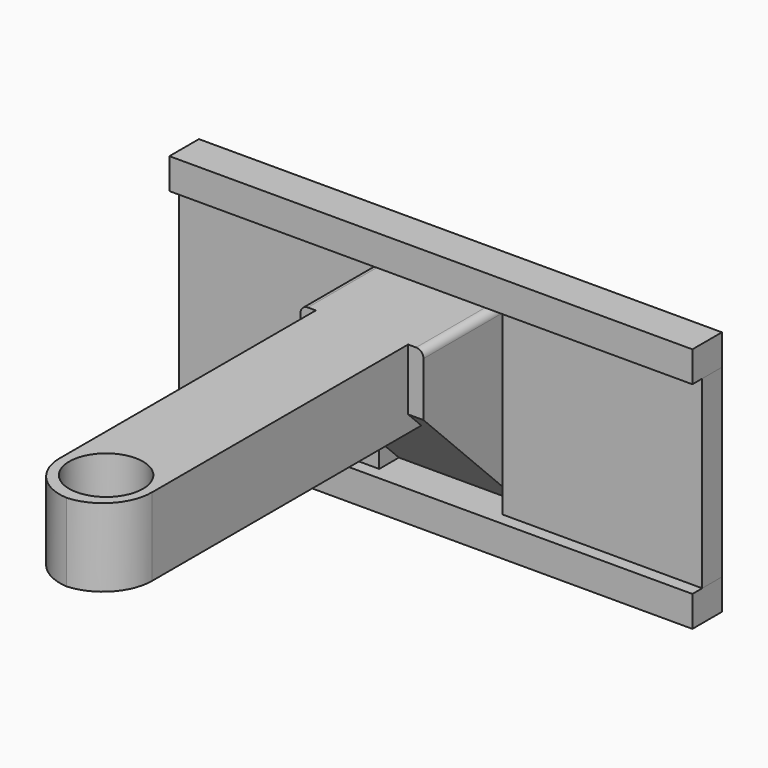
from build123d import *

# Parameters (mm, degrees)
F0_W         = 15.24
F0_H         = 12.7
F0_H_2       = 0.8601994222
F1_DEPTH     = 101.6
F2_DEPTH     = 25.4
F4_START     = 6.35
F3_R         = 7.62
F4_DEPTH     = 18.796
F5_T1_DEPTH  = 66.9001994222
F0_W_2       = 41.275
F0_H_3       = 38.1
F6_DEPTH     = 5.08
F0_W_3       = 107.95
F0_H_4       = 1.016
F0_H_5       = 4.318
F7_DEPTH     = 7.62
F8_R         = 1.524
F9_T4_DEPTH  = 156.0414957887
F9_T10_DEPTH = 156.0414957887
F9_T16_DEPTH = 156.0414957887
F9_T23_DEPTH = 156.0414957887
F9_T29_DEPTH = 156.0414957887


# Not quite as in the source:
# - a fillet or chamfer that OpenCascade refuses, or shapes differently, is made with other operations: its cross-section is extruded or revolved along the edge and cut away or added


with BuildPart() as f1:
    # F0 (on Front) → F1 (new body)
    with BuildSketch(Plane.XZ):
        Polygon((9.525, 2.9498005778), (9.525, 19.05), (7.62, 19.05), (7.62, 18.1898005778), (7.62, 5.4898005778), (-7.62, 5.4898005778), (-7.62, 18.1898005778), (-7.62, 19.05), (-9.525, 19.05), (-9.525, 2.9498005778), align=None)
        with Locations((0, 11.8398005778)):
            Rectangle(F0_W, F0_H)
        with Locations((0, 18.6199002889)):
            Rectangle(F0_W, F0_H_2)
    extrude(amount=F1_DEPTH)

    # F0 (on Front) → F2 (join)
    with BuildSketch(Plane.XZ):
        Polygon((12.7, -19.05), (12.7, 19.05), (9.525, 19.05), (9.525, 2.9498005778), (-9.525, 2.9498005778), (-9.525, 19.05), (-12.7, 19.05), (-12.7, -19.05), align=None)
    extrude(amount=F2_DEPTH)

    # F3 (on Top) → F4 (cut)
    with BuildSketch(Plane.XY.offset(F4_START)):
        with Locations((0, -91.4209560153)):
            Circle(F3_R)
    extrude(amount=F4_DEPTH, mode=Mode.SUBTRACT)

    # F5: fillet of radius 10.16 on 2 edges, made by hand

    # F5_s2 → F5_t1 (cut)
    with BuildSketch(Plane.XY.offset(-22.4501994222)):
        with BuildLine():
            ThreePointArc((9.525, -91.44), (6.5492048969, -98.6242048969), (-0.635, -101.6))
            Line((-0.635, -101.6), (9.525, -101.6))
            Line((9.525, -101.6), (9.525, -91.44))
        make_face()
        with BuildLine():
            ThreePointArc((0.635, -101.6), (-6.5492048969, -98.6242048969), (-9.525, -91.44))
            Line((-9.525, -91.44), (-9.525, -101.6))
            Line((-9.525, -101.6), (0.635, -101.6))
        make_face()
    extrude(amount=F5_T1_DEPTH, mode=Mode.SUBTRACT)

    # F8
    f8_edges = [f1.edges().sort_by_distance(p)[0] for p in [
        (-12.7, -12.7, 19.05),
        (12.7, -12.7, 19.05),
    ]]
    fillet(f8_edges, radius=F8_R)

    # F9: chamfer of 25.4 on 1 edges, made by hand


with BuildPart() as f6:
    # F0 (on Front) → F6 (new body)
    with BuildSketch(Plane.XZ):
        with Locations((-33.3375, 0)):
            Rectangle(F0_W_2, F0_H_3)
    extrude(amount=F6_DEPTH)


with BuildPart() as f6b:
    # F0 (on Front) → F6, piece 2 (new body)
    with BuildSketch(Plane.XZ):
        with Locations((33.3375, 0)):
            Rectangle(F0_W_2, F0_H_3)
    extrude(amount=F6_DEPTH)


with BuildPart() as f7:
    # F0 (on Front) → F7 (new body)
    with BuildSketch(Plane.XZ):
        Polygon((53.975, -20.066), (53.975, -19.05), (12.7, -19.05), (-12.7, -19.05), (-53.975, -19.05), (-53.975, -20.066), align=None)
        with Locations((0, -24.892)):
            Rectangle(F0_W_3, F0_H_4)
        with Locations((0, -22.225)):
            Rectangle(F0_W_3, F0_H_5)
    extrude(amount=F7_DEPTH)


with BuildPart() as f7b:
    # F0 (on Front) → F7, piece 2 (new body)
    with BuildSketch(Plane.XZ):
        with Locations((0, 22.225)):
            Rectangle(F0_W_3, F0_H_5)
        with Locations((0, 24.892)):
            Rectangle(F0_W_3, F0_H_4)
        Polygon((53.975, 19.05), (53.975, 20.066), (-53.975, 20.066), (-53.975, 19.05), (-12.7, 19.05), (-9.525, 19.05), (-7.62, 19.05), (7.62, 19.05), (9.525, 19.05), (12.7, 19.05), align=None)
    extrude(amount=F7_DEPTH)


with BuildPart() as f9_tool2:
    # F9_s3 → F9_t4 (new body)
    with BuildSketch(Plane.YZ.offset(-78.0207478943)):
        Polygon((-25.4, 6.35), (0, -19.05), (-25.4, -19.05), align=None)
    extrude(amount=F9_T4_DEPTH)

    split(bisect_by=Plane.XY.offset(2.9498005778), keep=Keep.TOP)

    split(bisect_by=Plane.YZ.offset(-9.525), keep=Keep.BOTTOM)


with BuildPart() as f1_1:
    add(f1.part)

    # F9_t1: cut F9_tool2
    add(f9_tool2.part, mode=Mode.SUBTRACT)


with BuildPart() as f9_tool8:
    # F9_s9 → F9_t10 (new body)
    with BuildSketch(Plane.YZ.offset(-78.0207478943)):
        Polygon((-25.4, 6.35), (0, -19.05), (-25.4, -19.05), align=None)
    extrude(amount=F9_T10_DEPTH)

    split(bisect_by=Plane.XY.offset(2.9498005778), keep=Keep.BOTTOM)

    split(bisect_by=Plane.YZ.offset(-9.525), keep=Keep.BOTTOM)


with BuildPart() as f1_2:
    add(f1_1.part)

    # F9_t7: cut F9_tool8
    add(f9_tool8.part, mode=Mode.SUBTRACT)


with BuildPart() as f9_tool14:
    # F9_s15 → F9_t16 (new body)
    with BuildSketch(Plane.YZ.offset(-78.0207478943)):
        Polygon((-25.4, 6.35), (0, -19.05), (-25.4, -19.05), align=None)
    extrude(amount=F9_T16_DEPTH)

    split(bisect_by=Plane.YZ.offset(9.525), keep=Keep.BOTTOM)

    split(bisect_by=Plane.XY.offset(2.9498005778), keep=Keep.BOTTOM)

    split(bisect_by=Plane.YZ.offset(-9.525), keep=Keep.TOP)


with BuildPart() as f1_3:
    add(f1_2.part)

    # F9_t13: cut F9_tool14
    add(f9_tool14.part, mode=Mode.SUBTRACT)


with BuildPart() as f9_tool21:
    # F9_s22 → F9_t23 (new body)
    with BuildSketch(Plane.YZ.offset(-78.0207478943)):
        Polygon((-25.4, 6.35), (0, -19.05), (-25.4, -19.05), align=None)
    extrude(amount=F9_T23_DEPTH)

    split(bisect_by=Plane.YZ.offset(9.525), keep=Keep.TOP)

    split(bisect_by=Plane.XY.offset(2.9498005778), keep=Keep.TOP)


with BuildPart() as f1_4:
    add(f1_3.part)

    # F9_t20: cut F9_tool21
    add(f9_tool21.part, mode=Mode.SUBTRACT)


with BuildPart() as f9_tool27:
    # F9_s28 → F9_t29 (new body)
    with BuildSketch(Plane.YZ.offset(-78.0207478943)):
        Polygon((-25.4, 6.35), (0, -19.05), (-25.4, -19.05), align=None)
    extrude(amount=F9_T29_DEPTH)

    split(bisect_by=Plane.YZ.offset(9.525), keep=Keep.TOP)

    split(bisect_by=Plane.XY.offset(2.9498005778), keep=Keep.BOTTOM)


with BuildPart() as f1_5:
    add(f1_4.part)

    # F9_t26: cut F9_tool27
    add(f9_tool27.part, mode=Mode.SUBTRACT)


solid = Compound([f6.part, f6b.part, f7.part, f7b.part, f1_5.part])
